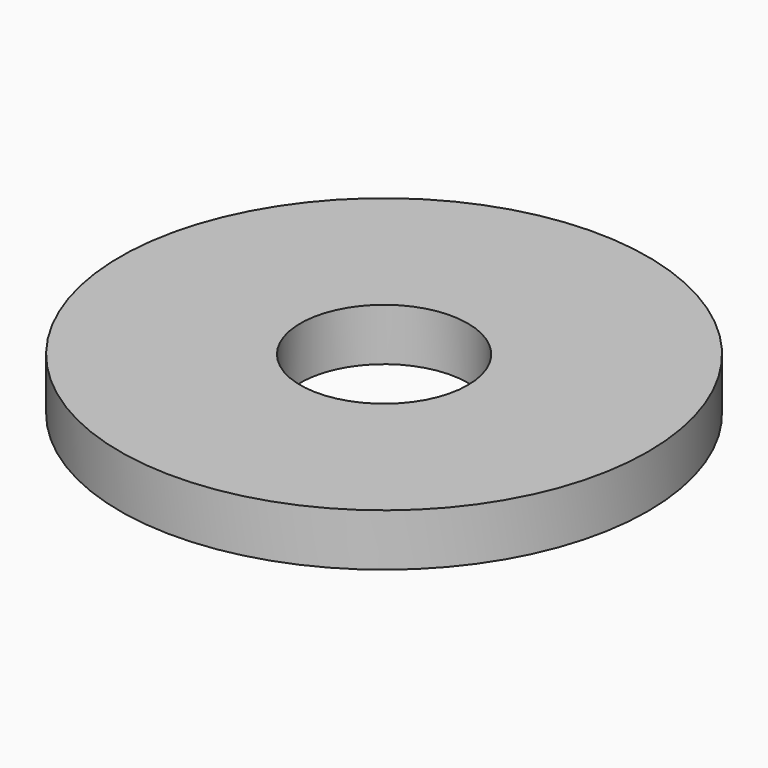
from build123d import *

# Parameters (mm, degrees)
F0_R     = 35.2425
F0_R_2   = 11.176
F1_DEPTH = 6.985
F2_DEPTH = 6.986


# Not quite as in the source:
# - a feature names something its author has since deleted; it is built from what else it names


with BuildPart() as f1:
    # F0 (on Top) → F1 (new body)
    with BuildSketch(Plane.XY):
        Circle(F0_R)
        Circle(F0_R_2, mode=Mode.SUBTRACT)
        Circle(F0_R_2)
    extrude(amount=F1_DEPTH)

    # F0 (on Top) → F2 (cut, through all)
    with BuildSketch(Plane.XY):
        Circle(F0_R_2)
    extrude(amount=F2_DEPTH, mode=Mode.SUBTRACT)


solid = f1.part
